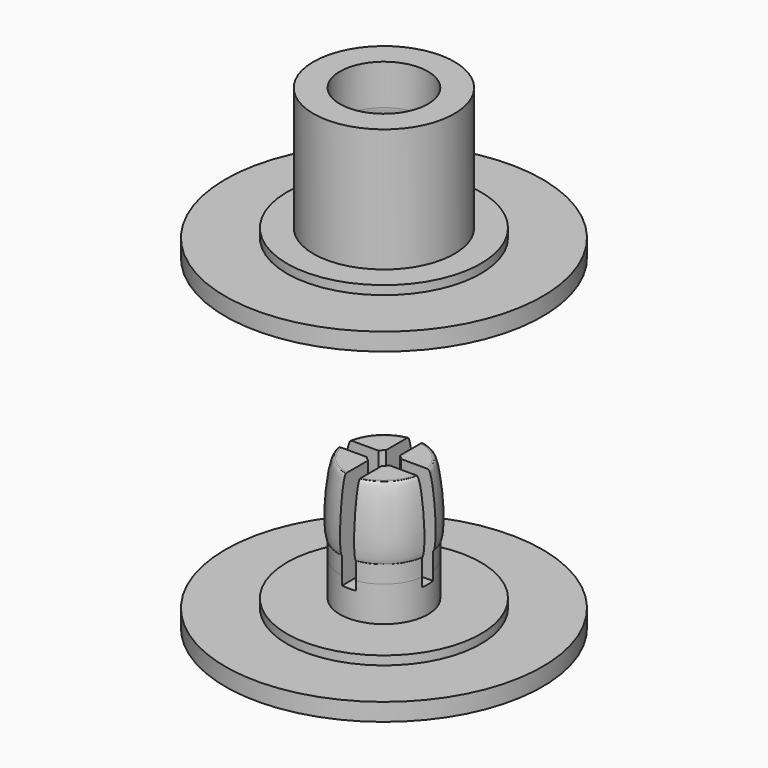
from build123d import *

# Parameters (mm, degrees)
F2_R     = 2
F4_W     = 0.8
F4_H     = 0.8
F5_DEPTH = 5.5


# Not quite as in the source:
# - ends of sketch curves that miss each other by under 0.0002 mm in the source are joined


with BuildPart() as f1:
    # F0 (on Front) → F1 (revolve)
    with BuildSketch(Plane.XZ):
        with BuildLine():
            Line((-9, 0), (0, 0))
            Line((0, 0), (0, 1.5))
            Line((0, 1.5), (-2.5, 1.5))
            add(Edge.make_bspline(
                [(-2.5, 5.5), (-3, 5.5), (-3, 3.5), (-3, 1.5), (-2.5, 1.5)],
                knots=[3.1415926536, 3.1415926536, 3.1415926536, 4.7123889804, 4.7123889804, 6.2831853072, 6.2831853072, 6.2831853072], degree=2, weights=[1, 0.7071067812, 1, 0.7071067812, 1]))
            Line((-2.5, 5.5), (-2.5, 8.5))
            Line((-2.5, 8.5), (-4, 8.5))
            Line((-4, 8.5), (-4, 1.5))
            Line((-4, 1.5), (-5.5, 1.5))
            Line((-5.5, 1.5), (-5.5, 1))
            Line((-5.5, 1), (-9, 1))
            Line((-9, 1), (-9, 0))
        make_face()
    revolve(axis=Axis((0, 0, 0.75), (0, 0, 1)))

    # F2
    f2_edges = [f1.edges().sort_by_distance(p)[0] for p in [
        (2.5, 0, 5.5),
    ]]
    fillet(f2_edges, radius=F2_R)


with BuildPart() as f3:
    # F0 (on Front) → F3 (revolve)
    with BuildSketch(Plane.XZ):
        with BuildLine():
            Line((-9, -18.5), (0, -18.5))
            Line((0, -18.5), (0, -17))
            Line((0, -17), (-0.75, -17))
            Line((-0.75, -17), (-0.75, -10))
            Line((-0.75, -10), (-2.14088, -10))
            Line((-2.14088, -10), (-2.2209772679, -10.009743799))
            add(Edge.make_bspline(
                [(-2.2209772679, -10.009743799), (-2.4703682805, -9.9923046805), (-2.609881228, -11.987432781), (-2.7493941755, -13.9825608816), (-2.5000031629, -14)],
                knots=[3.1415926536, 3.1415926536, 3.1415926536, 4.7123889804, 4.7123889804, 6.2831853072, 6.2831853072, 6.2831853072], degree=2, weights=[1, 0.7071067812, 1, 0.7071067812, 1]))
            Line((-2.5000031629, -14), (-2.5, -15))
            Line((-2.5, -15), (-2.5, -17))
            Line((-2.5, -17), (-4, -17))
            Line((-4, -17), (-5.5, -17))
            Line((-5.5, -17), (-5.5, -17.5))
            Line((-5.5, -17.5), (-9, -17.5))
            Line((-9, -17.5), (-9, -18.5))
        make_face()
    revolve(axis=Axis((0, 0, -17.75), (0, 0, -1)))

    # F4 (on face) → F5 (cut)
    with BuildSketch(Plane.XY.offset(-10)):
        with BuildLine():
            Line((-0.4, -6), (0.4, -6))
            Line((0.4, -6), (0.4, -2.1031802525))
            ThreePointArc((0.4, -2.1031802525), (0, -2.14088), (-0.4, -2.1031802525))
            Line((-0.4, -2.1031802525), (-0.4, -6))
        make_face()
        with BuildLine():
            ThreePointArc((-0.4, -2.1031802525), (0, -2.14088), (0.4, -2.1031802525))
            Line((0.4, -2.1031802525), (0.4, -0.634428877))
            ThreePointArc((0.4, -0.634428877), (0, -0.75), (-0.4, -0.634428877))
            Line((-0.4, -0.634428877), (-0.4, -2.1031802525))
        make_face()
        with BuildLine():
            ThreePointArc((-0.4, -0.634428877), (0, -0.75), (0.4, -0.634428877))
            Line((0.4, -0.634428877), (0.4, -0.4))
            Line((0.4, -0.4), (-0.4, -0.4))
            Line((-0.4, -0.4), (-0.4, -0.634428877))
        make_face()
        with BuildLine():
            Line((-0.634428877, -0.4), (-0.4, -0.4))
            Line((-0.4, -0.4), (-0.4, 0.4))
            Line((-0.4, 0.4), (-0.634428877, 0.4))
            ThreePointArc((-0.634428877, 0.4), (-0.75, 0), (-0.634428877, -0.4))
        make_face()
        with BuildLine():
            Line((-6, -0.4), (-2.1031802525, -0.4))
            ThreePointArc((-2.1031802525, -0.4), (-2.14088, 0), (-2.1031802525, 0.4))
            Line((-2.1031802525, 0.4), (-6, 0.4))
            Line((-6, 0.4), (-6, -0.4))
        make_face()
        Rectangle(F4_W, F4_H)
        with BuildLine():
            Line((-0.4, 0.4), (0.4, 0.4))
            Line((0.4, 0.4), (0.4, 0.634428877))
            ThreePointArc((0.4, 0.634428877), (0, 0.75), (-0.4, 0.634428877))
            Line((-0.4, 0.634428877), (-0.4, 0.4))
        make_face()
        with BuildLine():
            ThreePointArc((0.4, 2.1031802525), (0, 2.14088), (-0.4, 2.1031802525))
            Line((-0.4, 2.1031802525), (-0.4, 0.634428877))
            ThreePointArc((-0.4, 0.634428877), (0, 0.75), (0.4, 0.634428877))
            Line((0.4, 0.634428877), (0.4, 2.1031802525))
        make_face()
        with BuildLine():
            Line((-0.4, 6), (-0.4, 2.1031802525))
            ThreePointArc((-0.4, 2.1031802525), (0, 2.14088), (0.4, 2.1031802525))
            Line((0.4, 2.1031802525), (0.4, 6))
            Line((0.4, 6), (-0.4, 6))
        make_face()
        with BuildLine():
            Line((0.634428877, -0.4), (2.1031802525, -0.4))
            ThreePointArc((2.1031802525, -0.4), (2.1314342253, -0.2008863304), (2.14088, 0))
            ThreePointArc((2.14088, 0), (2.1314342253, 0.2008863304), (2.1031802525, 0.4))
            Line((2.1031802525, 0.4), (0.634428877, 0.4))
            ThreePointArc((0.634428877, 0.4), (0.7205281597, 0.2081806214), (0.75, 0))
            ThreePointArc((0.75, 0), (0.7205281597, -0.2081806214), (0.634428877, -0.4))
        make_face()
        with BuildLine():
            Line((0.4, 0.4), (0.4, -0.4))
            Line((0.4, -0.4), (0.634428877, -0.4))
            ThreePointArc((0.634428877, -0.4), (0.7205281597, -0.2081806214), (0.75, 0))
            ThreePointArc((0.75, 0), (0.7205281597, 0.2081806214), (0.634428877, 0.4))
            Line((0.634428877, 0.4), (0.4, 0.4))
        make_face()
        with BuildLine():
            ThreePointArc((2.14088, 0), (2.1314342253, -0.2008863304), (2.1031802525, -0.4))
            Line((2.1031802525, -0.4), (6, -0.4))
            Line((6, -0.4), (6, 0.4))
            Line((6, 0.4), (2.1031802525, 0.4))
            ThreePointArc((2.1031802525, 0.4), (2.1314342253, 0.2008863304), (2.14088, 0))
        make_face()
        with BuildLine():
            ThreePointArc((-2.1031802525, 0.4), (-2.14088, 0), (-2.1031802525, -0.4))
            Line((-2.1031802525, -0.4), (-0.634428877, -0.4))
            ThreePointArc((-0.634428877, -0.4), (-0.75, 0), (-0.634428877, 0.4))
            Line((-0.634428877, 0.4), (-2.1031802525, 0.4))
        make_face()
    extrude(amount=-F5_DEPTH, mode=Mode.SUBTRACT)


solid = Compound([f1.part, f3.part])
